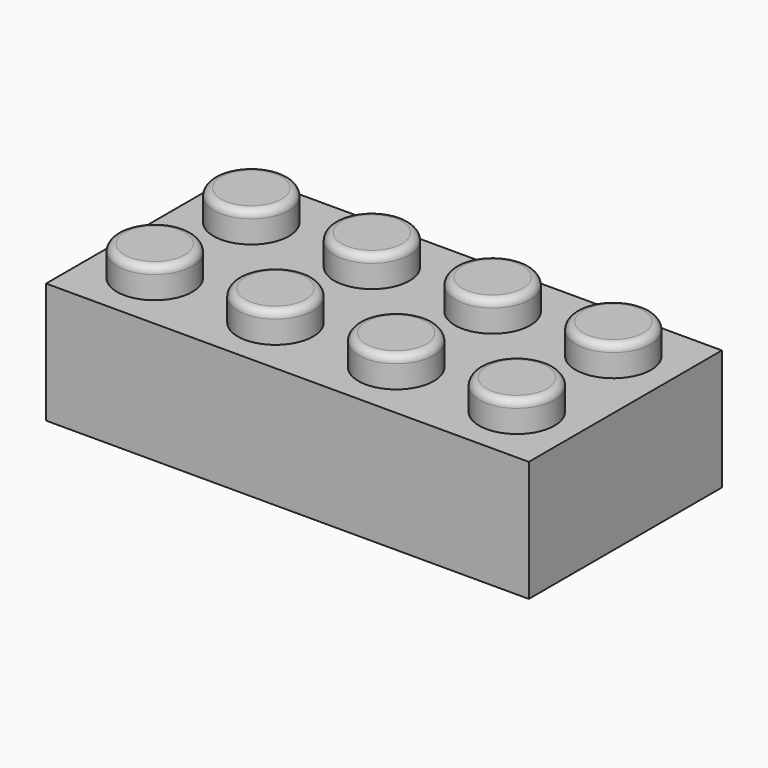
from build123d import *

# Parameters (mm, degrees)
F0_W        = 32
F0_H        = 16
F1_DEPTH    = 8
F2_R        = 2.5
F3_DEPTH    = 2
F4_R        = 0.5
F5_T        = -1.5
F6_R        = 3
F7_DEPTH    = 8
F8_T        = 1
F8_T3_DEPTH = 8.5
F8_T5_DEPTH = 15
F8_T7_DEPTH = 31


# Not quite as in the source:
# - a shell that OpenCascade refuses in one call is made with other operations: the cavity is built on its own and cut out


with BuildPart() as f1:
    # F0 (on Top) → F1 (new body)
    with BuildSketch(Plane.XY):
        with Locations((-1.4037434012, 1.4314407872)):
            Rectangle(F0_W, F0_H)
    extrude(amount=F1_DEPTH)

    # F2 (on face) → F3 (join)
    with BuildSketch(Plane.XY.offset(8)):
        with Locations((-13.4037434012, 5.4314407872)):
            Circle(F2_R)
        with Locations((-5.4037434012, 5.4314407872)):
            Circle(F2_R)
        with Locations((2.5962565988, 5.4314407872)):
            Circle(F2_R)
        with Locations((10.5962565988, 5.4314407872)):
            Circle(F2_R)
        with Locations((-13.4037434012, -2.5685592128)):
            Circle(F2_R)
        with Locations((-5.397730317, -2.5685592128)):
            Circle(F2_R)
        with Locations((2.602269683, -2.5685592128)):
            Circle(F2_R)
        with Locations((10.602269683, -2.5685592128)):
            Circle(F2_R)
    extrude(amount=F3_DEPTH)

    # F4
    f4_edges = [f1.edges().sort_by_distance(p)[0] for p in [
        (8.10227, -2.568559, 10),
        (8.096257, 5.431441, 10),
        (-15.903743, -2.568559, 10),
        (-7.89773, -2.568559, 10),
        (0.10227, -2.568559, 10),
        (0.096257, 5.431441, 10),
        (-7.903743, 5.431441, 10),
        (-15.903743, 5.431441, 10),
    ]]
    fillet(f4_edges, radius=F4_R)

    # F5
    f5_openings = [f1.faces().sort_by_distance(p)[0] for p in [
        (-1.403743, 1.431441, 0),
    ]]
    offset(amount=F5_T, openings=f5_openings, kind=Kind.INTERSECTION)

    # F6 (on face) → F7 (join)
    with BuildSketch(Plane(origin=(0, 0, 6.5), x_dir=(1, 0, 0), z_dir=(0, 0, -1))):
        with Locations((-9.3996422365, -1.4314407872)):
            Circle(F6_R)
        with Locations((-1.2057628483, -1.4314407872)):
            Circle(F6_R)
        with Locations((6.947263144, -1.4314407872)):
            Circle(F6_R)
    extrude(amount=F7_DEPTH)

    # F8: shell of thickness 1, made by hand


with BuildPart() as f8_core1:
    # F8_t2: copy of F1
    add(f1.part)

    # the walls: a layer under each face that stays
    f8_faces = [f8_core1.faces().sort_by_distance(p)[0] for p in [
        (-15.9037434012, -2.5685592128, 8.75),
        (-1.4037434012, 1.4314407872, 8),
        (-13.4037434012, -2.5685592128, 10),
        (14.5962565988, 1.4314407872, 4),
        (-1.4037434012, -6.5685592128, 4),
        (-1.4037434012, 9.4314407872, 4),
        (-17.4037434012, 1.4314407872, 4),
        (-7.897730317, -2.5685592128, 8.75),
        (0.102269683, -2.5685592128, 8.75),
        (8.102269683, -2.5685592128, 8.75),
        (-15.9037434012, 5.4314407872, 8.75),
        (-7.9037434012, 5.4314407872, 8.75),
        (0.0962565988, 5.4314407872, 8.75),
        (8.0962565988, 5.4314407872, 8.75),
        (-15.1180291155, -5.4257020699, 0),
        (13.0962565988, 1.4314407872, 3.25),
        (-1.4037434012, -5.0685592128, 3.25),
        (-15.9037434012, 1.4314407872, 3.25),
        (-1.4037434012, 7.9314407872, 3.25),
        (-5.397730317, -2.5685592128, 10),
        (2.602269683, -2.5685592128, 10),
        (10.602269683, -2.5685592128, 10),
        (-13.4037434012, 5.4314407872, 10),
        (-5.4037434012, 5.4314407872, 10),
        (2.5962565988, 5.4314407872, 10),
        (10.5962565988, 5.4314407872, 10),
        (-11.0704100678, -2.9018925461, 6.5),
        (-14.4037434012, -2.5685592128, 7.5),
        (-6.397730317, -2.5685592128, 7.5),
        (1.602269683, -2.5685592128, 7.5),
        (9.602269683, -2.5685592128, 7.5),
        (-12.3996422365, 1.4314407872, 2.5),
        (-14.4037434012, 5.4314407872, 7.5),
        (-6.4037434012, 5.4314407872, 7.5),
        (-4.2057628483, 1.4314407872, 2.5),
        (3.947263144, 1.4314407872, 2.5),
        (1.5962565988, 5.4314407872, 7.5),
        (9.5962565988, 5.4314407872, 7.5),
        (-13.4037434012, -2.5685592128, 8.5),
        (-5.397730317, -2.5685592128, 8.5),
        (2.602269683, -2.5685592128, 8.5),
        (10.602269683, -2.5685592128, 8.5),
        (-13.4037434012, 5.4314407872, 8.5),
        (-5.4037434012, 5.4314407872, 8.5),
        (2.5962565988, 5.4314407872, 8.5),
        (10.5962565988, 5.4314407872, 8.5),
    ]]
    thicken(f8_faces, amount=-F8_T, mode=Mode.SUBTRACT)

    # F8_s4 → F8_t3 (cut)
    with BuildSketch(Plane.XY.offset(-1)):
        Polygon((13.0862565988, -5.0585592128), (14.0962565988, -5.0685592128), (14.0962565988, -6.0685592128), (13.0962565988, -6.0685592128), align=None)
        Polygon((13.0862565988, 7.9214407872), (14.0962565988, 7.9314407872), (14.0962565988, 8.9314407872), (13.0962565988, 8.9314407872), align=None)
        Polygon((-15.8937434012, -5.0585592128), (-15.9037434012, -6.0685592128), (-16.9037434012, -6.0685592128), (-16.9037434012, -5.0685592128), align=None)
        Polygon((-15.8937434012, 7.9214407872), (-16.9037434012, 7.9314407872), (-16.9037434012, 8.9314407872), (-15.9037434012, 8.9314407872), align=None)
    extrude(amount=F8_T3_DEPTH, mode=Mode.SUBTRACT)

    # F8_s6 → F8_t5 (cut)
    with BuildSketch(Plane.XZ.offset(-8.9314407872)):
        Polygon((13.0862565988, 6.49), (14.0962565988, 6.5), (14.0962565988, 7.5), (13.0962565988, 7.5), align=None)
        Polygon((-15.8937434012, 6.49), (-16.9037434012, 6.5), (-16.9037434012, 7.5), (-15.9037434012, 7.5), align=None)
    extrude(amount=F8_T5_DEPTH, mode=Mode.SUBTRACT)

    # F8_s8 → F8_t7 (cut)
    with BuildSketch(Plane.YZ.offset(-16.9037434012)):
        Polygon((-5.0585592128, 6.49), (-6.0685592128, 6.5), (-6.0685592128, 7.5), (-5.0685592128, 7.5), align=None)
        Polygon((7.9214407872, 6.49), (8.9314407872, 6.5), (8.9314407872, 7.5), (7.9314407872, 7.5), align=None)
    extrude(amount=F8_T7_DEPTH, mode=Mode.SUBTRACT)

    # F8_s9 → F8_t10 (revolve, cut)
    with BuildSketch(Plane.XZ.offset(2.5685592128)):
        Polygon((-10.8937434012, 8.01), (-11.9037434012, 8), (-11.9037434012, 7), (-10.9037434012, 7), align=None)
    revolve(axis=Axis((-13.4037434012, -2.5685592128, 8), (0, 0, 1)), mode=Mode.SUBTRACT)

    # F8_s11 → F8_t12 (revolve, cut)
    with BuildSketch(Plane.XZ.offset(2.5685592128)):
        Polygon((-2.887730317, 8.01), (-2.897730317, 7), (-3.897730317, 7), (-3.897730317, 8), align=None)
    revolve(axis=Axis((-5.397730317, -2.5685592128, 8), (0, 0, 1)), mode=Mode.SUBTRACT)

    # F8_s13 → F8_t14 (revolve, cut)
    with BuildSketch(Plane.XZ.offset(2.5685592128)):
        Polygon((5.112269683, 8.01), (5.102269683, 7), (4.102269683, 7), (4.102269683, 8), align=None)
    revolve(axis=Axis((2.602269683, -2.5685592128, 8), (0, 0, 1)), mode=Mode.SUBTRACT)

    # F8_s15 → F8_t16 (revolve, cut)
    with BuildSketch(Plane.XZ.offset(2.5685592128)):
        Polygon((13.112269683, 8.01), (13.102269683, 7), (12.102269683, 7), (12.102269683, 8), align=None)
    revolve(axis=Axis((10.602269683, -2.5685592128, 8), (0, 0, 1)), mode=Mode.SUBTRACT)

    # F8_s17 → F8_t18 (revolve, cut)
    with BuildSketch(Plane.XZ.offset(-5.4314407872)):
        Polygon((-10.8937434012, 8.01), (-10.9037434012, 7), (-11.9037434012, 7), (-11.9037434012, 8), align=None)
    revolve(axis=Axis((-13.4037434012, 5.4314407872, 8), (0, 0, 1)), mode=Mode.SUBTRACT)

    # F8_s19 → F8_t20 (revolve, cut)
    with BuildSketch(Plane.XZ.offset(-5.4314407872)):
        Polygon((-2.8937434012, 8.01), (-2.9037434012, 7), (-3.9037434012, 7), (-3.9037434012, 8), align=None)
    revolve(axis=Axis((-5.4037434012, 5.4314407872, 8), (0, 0, 1)), mode=Mode.SUBTRACT)

    # F8_s21 → F8_t22 (revolve, cut)
    with BuildSketch(Plane.XZ.offset(-5.4314407872)):
        Polygon((5.1062565988, 8.01), (5.0962565988, 7), (4.0962565988, 7), (4.0962565988, 8), align=None)
    revolve(axis=Axis((2.5962565988, 5.4314407872, 8), (0, 0, 1)), mode=Mode.SUBTRACT)

    # F8_s23 → F8_t24 (revolve, cut)
    with BuildSketch(Plane.XZ.offset(-5.4314407872)):
        Polygon((13.1062565988, 8.01), (13.0962565988, 7), (12.0962565988, 7), (12.0962565988, 8), align=None)
    revolve(axis=Axis((10.5962565988, 5.4314407872, 8), (0, 0, 1)), mode=Mode.SUBTRACT)

    # F8_s25 → F8_t26 (revolve, cut)
    with BuildSketch(Plane.XZ.offset(-1.4314407872)):
        Polygon((-6.3896422365, 6.49), (-6.3996422365, 7.5), (-7.3996422365, 7.5), (-7.3996422365, 6.5), align=None)
    revolve(axis=Axis((-9.3996422365, 1.4314407872, 6.5), (0, 0, -1)), mode=Mode.SUBTRACT)

    # F8_s27 → F8_t28 (revolve, cut)
    with BuildSketch(Plane.XZ.offset(-1.4314407872)):
        Polygon((1.8042371517, 6.49), (1.7942371517, 7.5), (0.7942371517, 7.5), (0.7942371517, 6.5), align=None)
    revolve(axis=Axis((-1.2057628483, 1.4314407872, 6.5), (0, 0, -1)), mode=Mode.SUBTRACT)

    # F8_s29 → F8_t30 (revolve, cut)
    with BuildSketch(Plane.XZ.offset(-1.4314407872)):
        Polygon((9.957263144, 6.49), (9.947263144, 7.5), (8.947263144, 7.5), (8.947263144, 6.5), align=None)
    revolve(axis=Axis((6.947263144, 1.4314407872, 6.5), (0, 0, -1)), mode=Mode.SUBTRACT)

    # F8_s31 → F8_t32 (revolve, cut)
    with BuildSketch(Plane.XZ.offset(2.5685592128)):
        Polygon((-12.4137434012, 8.49), (-11.4037434012, 8.5), (-11.4037434012, 9.5), (-12.4037434012, 9.5), align=None)
    revolve(axis=Axis((-13.4037434012, -2.5685592128, 8.5), (0, 0, -1)), mode=Mode.SUBTRACT)

    # F8_s33 → F8_t34 (revolve, cut)
    with BuildSketch(Plane.XZ.offset(2.5685592128)):
        Polygon((-4.407730317, 8.49), (-3.397730317, 8.5), (-3.397730317, 9.5), (-4.397730317, 9.5), align=None)
    revolve(axis=Axis((-5.397730317, -2.5685592128, 8.5), (0, 0, -1)), mode=Mode.SUBTRACT)

    # F8_s35 → F8_t36 (revolve, cut)
    with BuildSketch(Plane.XZ.offset(2.5685592128)):
        Polygon((3.592269683, 8.49), (4.602269683, 8.5), (4.602269683, 9.5), (3.602269683, 9.5), align=None)
    revolve(axis=Axis((2.602269683, -2.5685592128, 8.5), (0, 0, -1)), mode=Mode.SUBTRACT)

    # F8_s37 → F8_t38 (revolve, cut)
    with BuildSketch(Plane.XZ.offset(2.5685592128)):
        Polygon((11.592269683, 8.49), (12.602269683, 8.5), (12.602269683, 9.5), (11.602269683, 9.5), align=None)
    revolve(axis=Axis((10.602269683, -2.5685592128, 8.5), (0, 0, -1)), mode=Mode.SUBTRACT)

    # F8_s39 → F8_t40 (revolve, cut)
    with BuildSketch(Plane.XZ.offset(-5.4314407872)):
        Polygon((-12.4137434012, 8.49), (-11.4037434012, 8.5), (-11.4037434012, 9.5), (-12.4037434012, 9.5), align=None)
    revolve(axis=Axis((-13.4037434012, 5.4314407872, 8.5), (0, 0, -1)), mode=Mode.SUBTRACT)

    # F8_s41 → F8_t42 (revolve, cut)
    with BuildSketch(Plane.XZ.offset(-5.4314407872)):
        Polygon((-4.4137434012, 8.49), (-3.4037434012, 8.5), (-3.4037434012, 9.5), (-4.4037434012, 9.5), align=None)
    revolve(axis=Axis((-5.4037434012, 5.4314407872, 8.5), (0, 0, -1)), mode=Mode.SUBTRACT)

    # F8_s43 → F8_t44 (revolve, cut)
    with BuildSketch(Plane.XZ.offset(-5.4314407872)):
        Polygon((3.5862565988, 8.49), (4.5962565988, 8.5), (4.5962565988, 9.5), (3.5962565988, 9.5), align=None)
    revolve(axis=Axis((2.5962565988, 5.4314407872, 8.5), (0, 0, -1)), mode=Mode.SUBTRACT)

    # F8_s45 → F8_t46 (revolve, cut)
    with BuildSketch(Plane.XZ.offset(-5.4314407872)):
        Polygon((11.5862565988, 8.49), (12.5962565988, 8.5), (12.5962565988, 9.5), (11.5962565988, 9.5), align=None)
    revolve(axis=Axis((10.5962565988, 5.4314407872, 8.5), (0, 0, -1)), mode=Mode.SUBTRACT)


with BuildPart() as f1_1:
    add(f1.part)

    # what is left inside the walls is the cavity
    f8_cavity = [f8_core1.part.solids().sort_by_distance(p)[0] for p in [
        (4.957263, 1.431441, 4.166667),
        (-11.389642, 1.431441, 4.166667),
        (-3.195763, 1.431441, 4.166667),
    ]]
    add(f8_cavity, mode=Mode.SUBTRACT)


solid = f1_1.part
